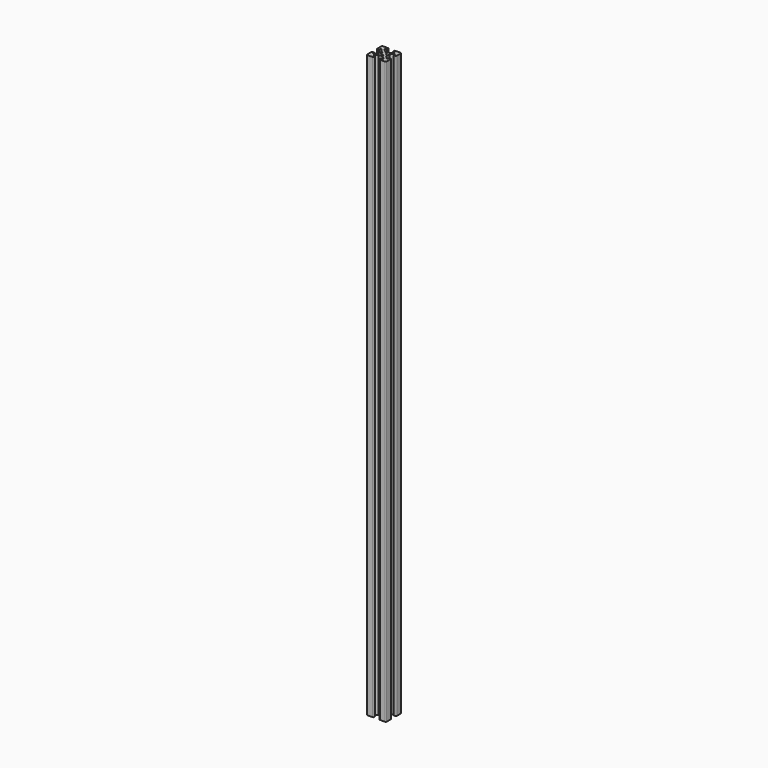
from build123d import *

# Parameters (mm, degrees)
F1_DEPTH = 600
F2_R     = 1
F3_R     = 0.5
F4_R     = 0.1


with BuildPart() as f1:
    # F0 (on Top) → F1 (new body)
    with BuildSketch(Plane.XY):
        with BuildLine():
            Line((-0.025, 4.0583112277), (-2.2905442747, 4.0583112277))
            Line((-2.2905442747, 4.0583112277), (-5.8640526549, 7.6318196079))
            Line((-5.8640526549, 7.6318196079), (-3, 7.6318196079))
            Line((-3, 7.6318196079), (-3, 10))
            Line((-3, 10), (-10, 10))
            Line((-10, 10), (-10, 3))
            Line((-10, 3), (-7.6318196079, 3))
            Line((-7.6318196079, 3), (-7.6318196079, 5.8640526549))
            Line((-7.6318196079, 5.8640526549), (-4, 2.232233047))
            Line((-4, 2.232233047), (-4, 0.025))
            Line((-4, 0.025), (-2.8230957687, 0.025))
            Line((-2.8230957687, 0.025), (-2.8230957687, 0.7926485917))
            Line((-2.8230957687, 0.7926485917), (-1.8740334308, 1.411684829))
            ThreePointArc((-1.8740334308, 1.411684829), (-2.3460869309, 0.0270456781), (-1.906078865, -1.3681077138))
            Line((-1.906078865, -1.3681077138), (-2.8238623803, -0.7794121329))
            Line((-2.8238623803, -0.7794121329), (-2.8238623803, -0.025))
            Line((-2.8238623803, -0.025), (-4, -0.025))
            Line((-4, -0.025), (-4, -2.232233047))
            Line((-4, -2.232233047), (-7.6318196079, -5.8640526549))
            Line((-7.6318196079, -5.8640526549), (-7.6318196079, -3))
            Line((-7.6318196079, -3), (-10, -3))
            Line((-10, -3), (-10, -10))
            Line((-10, -10), (-3, -10))
            Line((-3, -10), (-3, -7.6318196079))
            Line((-3, -7.6318196079), (-5.8640526549, -7.6318196079))
            Line((-5.8640526549, -7.6318196079), (-2.232233047, -4))
            Line((-2.232233047, -4), (-0.05, -4))
            Line((-0.05, -4), (-0.05, -2.9588690959))
            Line((-0.05, -2.9588690959), (-0.7483266194, -2.9588690959))
            Line((-0.7483266194, -2.9588690959), (-1.5537911294, -1.7580069631))
            ThreePointArc((-1.5537911294, -1.7580069631), (-0.0257632285, -2.3461013645), (1.5148107083, -1.7917041816))
            Line((1.5148107083, -1.7917041816), (0.7406048023, -2.9588690959))
            Line((0.7406048023, -2.9588690959), (0.05, -2.9588690959))
            Line((0.05, -2.9588690959), (0.05, -4))
            Line((0.05, -4), (2.232233047, -4))
            Line((2.232233047, -4), (5.8640526549, -7.6318196079))
            Line((5.8640526549, -7.6318196079), (3, -7.6318196079))
            Line((3, -7.6318196079), (3, -10))
            Line((3, -10), (10, -10))
            Line((10, -10), (10, -3))
            Line((10, -3), (7.6318196079, -3))
            Line((7.6318196079, -3), (7.6318196079, -5.8640526549))
            Line((7.6318196079, -5.8640526549), (4, -2.232233047))
            Line((4, -2.232233047), (4, -0.025))
            Line((4, -0.025), (2.8238623803, -0.025))
            Line((2.8238623803, -0.025), (2.8238623803, -0.7921485609))
            Line((2.8238623803, -0.7921485609), (1.8740334308, -1.411684829))
            ThreePointArc((1.8740334308, -1.411684829), (2.3460040432, 0.0334721598), (1.8329957125, 1.4645757318))
            Line((1.8329957125, 1.4645757318), (2.8230957687, 0.8068363719))
            Line((2.8230957687, 0.8068363719), (2.8230957687, 0.025))
            Line((2.8230957687, 0.025), (4, 0.025))
            Line((4, 0.025), (4, 2.232233047))
            Line((4, 2.232233047), (7.6318196079, 5.8640526549))
            Line((7.6318196079, 5.8640526549), (7.6318196079, 3))
            Line((7.6318196079, 3), (10, 3))
            Line((10, 3), (10, 10))
            Line((10, 10), (3, 10))
            Line((3, 10), (3, 7.6318196079))
            Line((3, 7.6318196079), (5.8640526549, 7.6318196079))
            Line((5.8640526549, 7.6318196079), (2.2905442747, 4.0583112277))
            Line((2.2905442747, 4.0583112277), (0.025, 4.0583112277))
            Line((0.025, 4.0583112277), (0.025, 2.9460287187))
            Line((0.025, 2.9460287187), (0.7554459771, 2.9460287187))
            Line((0.7554459771, 2.9460287187), (1.5118729288, 1.7941838266))
            ThreePointArc((1.5118729288, 1.7941838266), (-0.0195250931, 2.3461615731), (-1.5415243666, 1.7687730164))
            Line((-1.5415243666, 1.7687730164), (-0.7608180556, 2.9474266339))
            Line((-0.7608180556, 2.9474266339), (-0.025, 2.9474266339))
            Line((-0.025, 2.9474266339), (-0.025, 4.0583112277))
        make_face()
    extrude(amount=F1_DEPTH)

    # F2
    f2_edges = [f1.edges().sort_by_distance(p)[0] for p in [
        (10, 10, 300),
        (10, -10, 300),
        (-10, -10, 300),
        (-3, -10, 300),
        (3, -10, 300),
        (-3, 10, 300),
        (-10, 3, 300),
        (10, 3, 300),
        (10, -3, 300),
        (-10, -3, 300),
        (-10, 10, 300),
        (3, 10, 300),
    ]]
    fillet(f2_edges, radius=F2_R)

    # F3
    f3_edges = [f1.edges().sort_by_distance(p)[0] for p in [
        (-7.63182, 5.864053, 300),
        (-5.864053, 7.63182, 300),
        (5.864053, 7.63182, 300),
        (7.63182, 5.864053, 300),
        (-7.63182, -5.864053, 300),
        (-5.864053, -7.63182, 300),
        (5.864053, -7.63182, 300),
        (7.63182, -5.864053, 300),
    ]]
    fillet(f3_edges, radius=F3_R)

    # F4
    f4_edges = [f1.edges().sort_by_distance(p)[0] for p in [
        (-1.874033, 1.411685, 300),
        (2.290544, 4.058311, 300),
        (4.656946, 7.63182, 300),
        (-1.541524, 1.768773, 300),
        (1.514811, -1.791704, 300),
        (1.874033, -1.411685, 300),
        (1.832996, 1.464576, 300),
        (1.511873, 1.794184, 300),
        (-1.906079, -1.368108, 300),
        (-1.553791, -1.758007, 300),
    ]]
    fillet(f4_edges, radius=F4_R)


solid = f1.part
